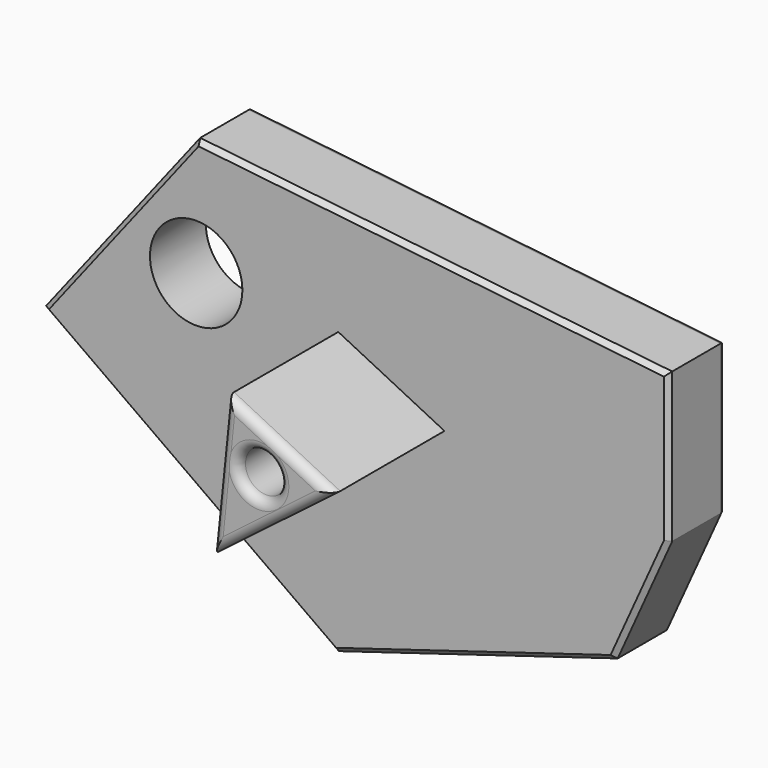
from build123d import *

# Parameters (mm, degrees)
F1_DEPTH     = 76.2
F2_SIZE      = 5.08
F4_DEPTH     = 152.4
F5_R         = 50.4680515056
F6_DEPTH     = 76.2
F7_R         = 22.662684834
F8_DEPTH     = 228.6
F9_R         = 5.08
F10_T1_DEPTH = 217.1500590573
F10_T3_DEPTH = 210.0843614146
F10_T5_DEPTH = 180.2491648874


# Not quite as in the source:
# - a fillet or chamfer that OpenCascade refuses, or shapes differently, is made with other operations: its cross-section is extruded or revolved along the edge and cut away or added


with BuildPart() as f1:
    # F0 (on Front) → F1 (new body)
    with BuildSketch(Plane.XZ):
        Polygon((376.9832551479, 180.0154298544), (-138.5454237461, 237.0085567236), (-306.9341778755, 20.6937491894), (13.0044706166, -207.2787433863), (317.3995614052, -115.3125613928), (376.9832551479, 16.8078560382), align=None)
    extrude(amount=F1_DEPTH)

    # F2
    f2_edges = [f1.edges().sort_by_distance(p)[0] for p in [
        (-146.964854, -76.2, -93.292497),
        (165.202016, -76.2, -161.295652),
        (347.191408, -76.2, -49.252353),
        (376.983255, -76.2, 98.411643),
        (119.218916, -76.2, 208.511993),
        (-222.739801, -76.2, 128.851153),
    ]]
    chamfer(f2_edges, length=F2_SIZE)

    # F3 (on face) → F4 (join)
    with BuildSketch(Plane.XZ.offset(76.2)):
        Polygon((132.2494894266, 45.2478192747), (16.2920933217, 102.7888357639), (0, -55.6601323187), align=None)
    extrude(amount=F4_DEPTH)

    # F5 (on face) → F6 (cut)
    with BuildSketch(Plane.XZ.offset(76.2)):
        with Locations((-138.9218121767, 108.8546961546)):
            Circle(F5_R)
    extrude(amount=-F6_DEPTH, mode=Mode.SUBTRACT)

    # F7 (on face) → F8 (cut)
    with BuildSketch(Plane.XZ.offset(228.6)):
        with Locations((51.4107942581, 38.0054563284)):
            Circle(F7_R)
    extrude(amount=-F8_DEPTH, mode=Mode.SUBTRACT)

    # F9
    f9_edges = [f1.edges().sort_by_distance(p)[0] for p in [
        (-146.964854, 0, -93.292497),
        (165.202016, 0, -161.295652),
        (347.191408, 0, -49.252353),
        (376.983255, 0, 98.411643),
        (119.218916, 0, 208.511993),
        (-222.739801, 0, 128.851153),
    ]]
    fillet(f9_edges, radius=F9_R)

    # F10: fillet of radius 10.16 on 4 edges, made by hand

    # F10_s2 → F10_t1 (cut)
    with BuildSketch(Plane(origin=(-47.0353574765, 0, -35.8885436609), x_dir=(0, 1, 0), z_dir=(0.7950071685, 0, 0.6066000347))):
        with BuildLine():
            ThreePointArc((-218.44, -44.2502041916), (-225.6242048969, -41.2744090884), (-228.6, -34.0902041916))
            Line((-228.6, -34.0902041916), (-228.6, -44.2502041916))
            Line((-228.6, -44.2502041916), (-218.44, -44.2502041916))
        make_face()
    extrude(amount=F10_T1_DEPTH, mode=Mode.SUBTRACT)

    # F10_s4 → F10_t3 (cut)
    with BuildSketch(Plane(origin=(13.2268524744, 0, 128.6379278687), x_dir=(0, 1, 0), z_dir=(-0.102283069, 0, -0.9947553336))):
        with BuildLine():
            ThreePointArc((-218.44, 5.6930891519), (-225.6242048969, 8.668884255), (-228.6, 15.8530891519))
            Line((-228.6, 15.8530891519), (-228.6, 5.6930891519))
            Line((-228.6, 5.6930891519), (-218.44, 5.6930891519))
        make_face()
    extrude(amount=F10_T3_DEPTH, mode=Mode.SUBTRACT)

    # F10_s6 → F10_t5 (cut)
    with BuildSketch(Plane(origin=(110.8548223357, 0, -55.0089892857), x_dir=(0, 1, 0), z_dir=(-0.8957755441, 0, 0.4445066644))):
        with BuildLine():
            ThreePointArc((-218.44, -99.3176693375), (-225.6242048969, -96.3418742344), (-228.6, -89.1576693375))
            Line((-228.6, -89.1576693375), (-228.6, -99.3176693375))
            Line((-228.6, -99.3176693375), (-218.44, -99.3176693375))
        make_face()
    extrude(amount=F10_T5_DEPTH, mode=Mode.SUBTRACT)

    # F10_s7 → F10_t8 (revolve, cut)
    with BuildSketch(Plane.XY.offset(38.0054563284)):
        with BuildLine():
            ThreePointArc((74.0734790921, -218.44), (77.0492741953, -225.6242048969), (84.2334790921, -228.6))
            Line((84.2334790921, -228.6), (74.0734790921, -228.6))
            Line((74.0734790921, -228.6), (74.0734790921, -218.44))
        make_face()
    revolve(axis=Axis((51.4107942581, -228.6, 38.0054563284), (0, -1, 0)), mode=Mode.SUBTRACT)


solid = f1.part
